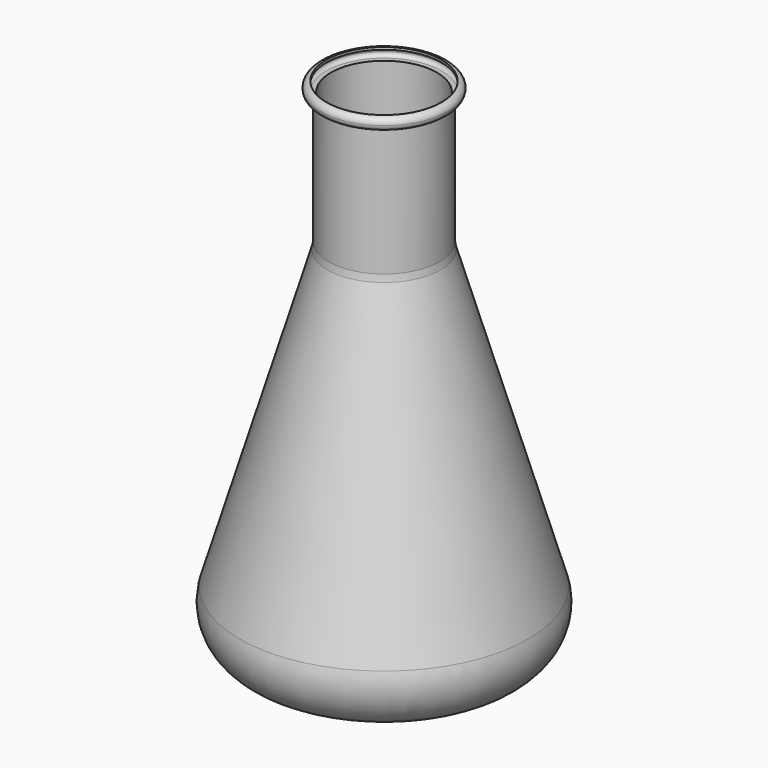
from build123d import *

# Parameters (mm, degrees)
F1_R      = 64
F2_DEPTH  = 55
F2_TAPER  = 16.5
F3_R      = 66.5
F4_DEPTH  = 148
F4_TAPER  = 16.5
F5_R      = 20
F6_R      = 20
F7_R      = 22.6604027456
F8_DEPTH  = 54
F9_R      = 26
F10_DEPTH = 5
F11_R     = 2.49999
F12_T     = -1
F13_R     = 10


# Not quite as in the source:
# - a fillet or chamfer is up to 0.001 mm smaller than in the source, because OpenCascade refuses the exact size
# - a shell that OpenCascade refuses in one call is made with other operations: the cavity is built on its own and cut out


with BuildPart() as f2:
    # F1 (on offset) → F2 (new body)
    with BuildSketch(Plane.XY.offset(4)):
        Circle(F1_R)
    extrude(amount=F2_DEPTH, taper=F2_TAPER)

    # F6
    f6_edges = [f2.edges().sort_by_distance(p)[0] for p in [
        (-64, 0, 4),
    ]]
    fillet(f6_edges, radius=F6_R)


with BuildPart() as f4:
    # F3 (on Top) → F4 (new body)
    with BuildSketch(Plane.XY):
        Circle(F3_R)
    extrude(amount=F4_DEPTH, taper=F4_TAPER)

    # F5
    f5_edges = [f4.edges().sort_by_distance(p)[0] for p in [
        (-66.5, 0, 0),
    ]]
    fillet(f5_edges, radius=F5_R)

    # F7 (on face) → F8 (join)
    with BuildSketch(Plane.XY.offset(148)):
        Circle(F7_R)
    extrude(amount=F8_DEPTH)

    # F9 (on face) → F10 (join)
    with BuildSketch(Plane.XY.offset(202)):
        Circle(F9_R)
    extrude(amount=F10_DEPTH)

    # F11 (radius 2.5 in the source; OpenCascade refuses exactly that, so slightly less here)
    f11_edges = [f4.edges().sort_by_distance(p)[0] for p in [
        (-26, 0, 207),
        (-26, 0, 202),
    ]]
    fillet(f11_edges, radius=F11_R)

    # F12: a shell. OpenCascade refuses it in one call, so the cavity is built on its own and cut out:
    # the body offset inwards by the wall thickness, plus a prism from it out through each open face.
    f12_core = offset(f4.part, amount=F12_T, kind=Kind.INTERSECTION, mode=Mode.PRIVATE)
    f12_exits = [f12_core.faces().sort_by_distance(p)[0] for p in [
        (0, 0, 206),
    ]]
    add(f12_core, mode=Mode.SUBTRACT)
    extrude(f12_exits, amount=-F12_T, mode=Mode.SUBTRACT)

    # F13
    f13_edges = [f4.edges().sort_by_distance(p)[0] for p in [
        (-22.660403, 0, 148),
    ]]
    fillet(f13_edges, radius=F13_R)


solid = Compound([f2.part, f4.part])
